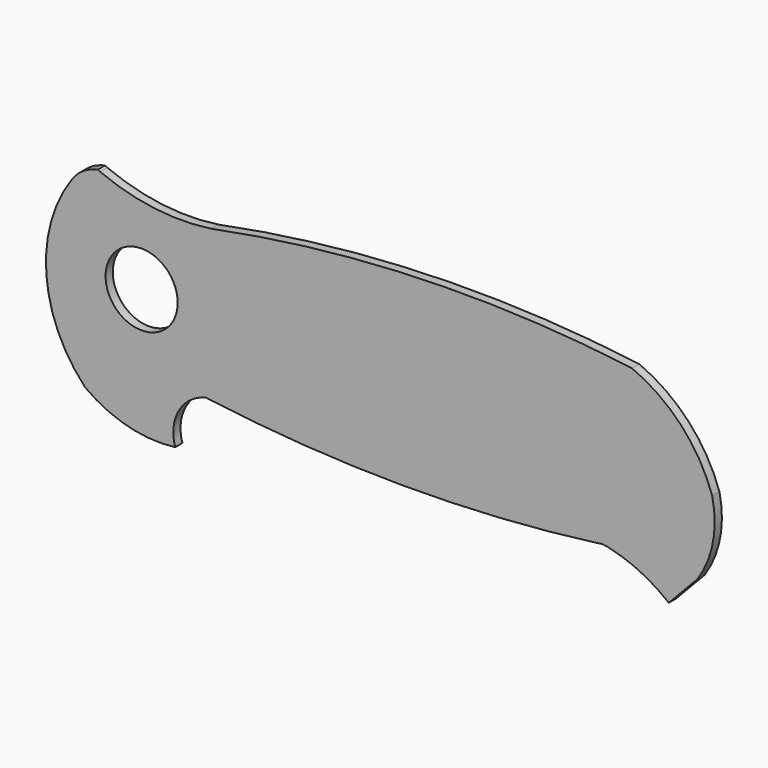
from build123d import *

# Parameters (mm, degrees)
F0_R     = 10
F1_DEPTH = 2.5


# Not quite as in the source:
# - a feature names something its author has since deleted; it is built from what else it names


with BuildPart() as f1:
    # F0 (on Front) → F1 (new body)
    with BuildSketch(Plane.XZ):
        with BuildLine():
            ThreePointArc((3.5229699651, 0.2896982716), (2.9467535756, 0.1596707418), (2.3780377062, 0))
            Line((2.3780377062, 0), (4.205058077, 0))
            ThreePointArc((4.205058077, 0), (3.8635532968, 0.1437643709), (3.5229699651, 0.2896982716))
        make_face()
        with BuildLine():
            Line((4.205058077, 0), (2.3780377062, 0))
            ThreePointArc((2.3780377062, 0), (-0.903638288, -1.6292874632), (-3.4998361796, -4.2145788348))
            ThreePointArc((-3.4998361796, -4.2145788348), (-3.5325783371, -4.260242238), (-3.5652547335, -4.3059527224))
            ThreePointArc((-3.5652547335, -4.3059527224), (-10.7285361122, -29.7799444124), (0, -53.9695158351))
            ThreePointArc((0, -53.9695158351), (11.8831829855, -59.6411390335), (25.0231431088, -60.4889571322))
            ThreePointArc((25.0231431088, -60.4889571322), (26.0566140951, -51.1714178585), (33.5999478712, -45.6052058665))
            ThreePointArc((33.5999478712, -45.6052058665), (87.8201274571, -49.2962363), (142.0548581476, -45.8255638994))
            ThreePointArc((142.0548581476, -45.8255638994), (142.7021149729, -45.7037001136), (143.3588035872, -45.6531803752))
            ThreePointArc((143.3588035872, -45.6531803752), (143.5374590966, -45.629232164), (143.7161041215, -45.6052058665))
            ThreePointArc((143.7161041215, -45.6052058665), (143.95071498, -45.6477329831), (144.1850665045, -45.6916667233))
            ThreePointArc((144.1850665045, -45.6916667233), (144.6977602251, -45.7735054296), (145.2015099012, -45.899158479))
            ThreePointArc((145.2015099012, -45.899158479), (154.032538738, -48.9458086752), (161.9085475054, -53.9695158351))
            Line((161.9085475054, -53.9695158351), (169.8591839037, -45.6052058665))
            ThreePointArc((169.8591839037, -45.6052058665), (174.1858351689, -35.1766319754), (173.9545511242, -23.8885155575))
            ThreePointArc((173.9545511242, -23.8885155575), (165.4122565919, -9.5597842761), (151.7413436521, 0))
            ThreePointArc((151.7413436521, 0), (93.1999930381, 2.7960741366), (34.9746532738, -3.8910456933))
            ThreePointArc((34.9746532738, -3.8910456933), (19.3261135001, -4.0311421401), (4.205058077, 0))
        make_face()
        with Locations((15.7105848193, -25)):
            Circle(F0_R, mode=Mode.SUBTRACT)
    extrude(amount=F1_DEPTH)


solid = f1.part
